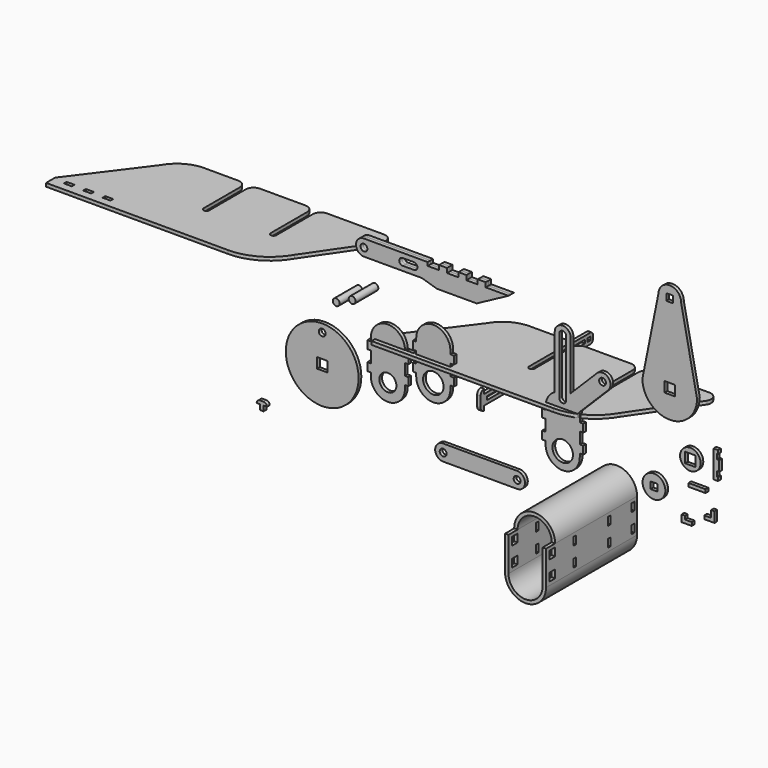
from build123d import *

# Parameters (mm, degrees)
F3_W      = 7
F3_H      = 3
F4_DEPTH  = 3
F2_W      = 7
F2_H      = 3
F5_DEPTH  = 3
F0_R      = 3
F6_DEPTH  = 3
F7_DEPTH  = 3
F8_R      = 9
F8_R_2    = 3
F9_DEPTH  = 3
F10_R     = 3
F11_DEPTH = 25
F12_R     = 3
F13_DEPTH = 25
F14_R     = 32
F14_W     = 9
F14_H     = 9
F14_R_2   = 3
F15_DEPTH = 3
F16_R     = 3
F17_DEPTH = 3
F18_R     = 10
F19_DEPTH = 100
F21_DEPTH = 100
F22_W     = 10
F22_H     = 18
F22_W_2   = 6
F22_H_2   = 7
F22_W_3   = 3
F23_DEPTH = 549.1479035941
F24_R     = 9
F25_DEPTH = 3
F1_R      = 7.5
F26_DEPTH = 3
F27_W     = 21
F27_H     = 3
F27_W_2   = 6
F27_W_3   = 18
F27_W_4   = 3
F28_DEPTH = 3
F29_R     = 3
F30_W     = 9
F30_H     = 9
F30_W_2   = 6
F30_H_2   = 6
F31_DEPTH = 3
F32_R     = 9
F32_W     = 9
F32_H     = 9
F33_DEPTH = 3
F35_DEPTH = 3
F36_DEPTH = 9
F38_DEPTH = 3
F40_W     = 3
F40_H     = 3
F41_DEPTH = 3
F43_DEPTH = 3
F45_DEPTH = 3
F46_W     = 15
F46_H     = 3
F47_DEPTH = 3
F48_R     = 10
F48_W     = 6
F48_H     = 6
F49_DEPTH = 3


# Not quite as in the source:
# - a feature names something its author has since deleted; it is built from what else it names


with BuildPart() as f4:
    # F3 (on Top) → F4 (new body)
    with BuildSketch(Plane.XY):
        with BuildLine():
            Line((-372.4580572146, 47.2241180668), (-372.4580572146, 37.2241180668))
            Line((-372.4580572146, 37.2241180668), (-212.4580572146, 37.2241180668))
            ThreePointArc((-212.4580572146, 37.2241180668), (-189.4580572146, 43.3869494928), (-172.6208886405, 60.2241180668))
            Line((-172.6208886405, 60.2241180668), (-137.4151172746, 111.7241180668))
            ThreePointArc((-137.4151172746, 111.7241180668), (-137.4151172746, 118.7241180668), (-143.4772951011, 122.2241180668))
            Line((-143.4772951011, 122.2241180668), (-193.4772951011, 122.2241180668))
            ThreePointArc((-193.4772951011, 122.2241180668), (-198.4270425694, 120.1738655351), (-200.4772951011, 115.2241180668))
            Line((-200.4772951011, 115.2241180668), (-200.4772951011, 75.2241180668))
            ThreePointArc((-200.4772951011, 75.2241180668), (-202.9772951011, 72.7241180668), (-205.4772951011, 75.2241180668))
            Line((-205.4772951011, 75.2241180668), (-205.4772951011, 115.2241180668))
            ThreePointArc((-205.4772951011, 115.2241180668), (-207.5275476328, 120.1738655351), (-212.4772951011, 122.2241180668))
            Line((-212.4772951011, 122.2241180668), (-252.4772951011, 122.2241180668))
            ThreePointArc((-252.4772951011, 122.2241180668), (-257.4270425694, 120.1738655351), (-259.4772951011, 115.2241180668))
            Line((-259.4772951011, 115.2241180668), (-259.4772951011, 75.2241180668))
            ThreePointArc((-259.4772951011, 75.2241180668), (-261.9772951011, 72.7241180668), (-264.4772951011, 75.2241180668))
            Line((-264.4772951011, 75.2241180668), (-264.4772951011, 115.2241180668))
            ThreePointArc((-264.4772951011, 115.2241180668), (-266.5275476328, 120.1738655351), (-271.4772951011, 122.2241180668))
            Line((-271.4772951011, 122.2241180668), (-301.4772951011, 122.2241180668))
            ThreePointArc((-301.4772951011, 122.2241180668), (-316.4772951011, 118.2048801804), (-327.4580572146, 107.2241180668))
            Line((-327.4580572146, 107.2241180668), (-372.4580572146, 47.2241180668))
        make_face()
        with Locations((-358.9580572146, 45.7241180668)):
            Rectangle(F3_W, F3_H, mode=Mode.SUBTRACT)
        with Locations((-341.9580572146, 45.7241180668)):
            Rectangle(F3_W, F3_H, mode=Mode.SUBTRACT)
        with Locations((-324.9580572146, 45.7241180668)):
            Rectangle(F3_W, F3_H, mode=Mode.SUBTRACT)
    extrude(amount=F4_DEPTH)


with BuildPart() as f5:
    # F2 (on Top) → F5 (new body)
    with BuildSketch(Plane.XY):
        with BuildLine():
            Line((-51.2112602569, 3.1967771862), (-51.2112602569, -6.8032228138))
            Line((-51.2112602569, -6.8032228138), (108.7887397431, -6.8032228138))
            ThreePointArc((108.7887397431, -6.8032228138), (131.7887397431, -0.6403913879), (148.6259083172, 16.1967771862))
            Line((148.6259083172, 16.1967771862), (183.8316796831, 67.6967771862))
            ThreePointArc((183.8316796831, 67.6967771862), (183.8316796831, 74.6967771862), (177.7695018566, 78.1967771862))
            Line((177.7695018566, 78.1967771862), (127.7695018566, 78.1967771862))
            ThreePointArc((127.7695018566, 78.1967771862), (122.8197543883, 76.1465246545), (120.7695018566, 71.1967771862))
            Line((120.7695018566, 71.1967771862), (120.7695018566, 31.1967771862))
            ThreePointArc((120.7695018566, 31.1967771862), (118.2695018566, 28.6967771862), (115.7695018566, 31.1967771862))
            Line((115.7695018566, 31.1967771862), (115.7695018566, 71.1967771862))
            ThreePointArc((115.7695018566, 71.1967771862), (113.7192493249, 76.1465246545), (108.7695018566, 78.1967771862))
            Line((108.7695018566, 78.1967771862), (68.7695018566, 78.1967771862))
            ThreePointArc((68.7695018566, 78.1967771862), (63.8197543883, 76.1465246545), (61.7695018566, 71.1967771862))
            Line((61.7695018566, 71.1967771862), (61.7695018566, 31.1967771862))
            ThreePointArc((61.7695018566, 31.1967771862), (59.2695018566, 28.6967771862), (56.7695018566, 31.1967771862))
            Line((56.7695018566, 31.1967771862), (56.7695018566, 71.1967771862))
            ThreePointArc((56.7695018566, 71.1967771862), (54.7192493249, 76.1465246545), (49.7695018566, 78.1967771862))
            Line((49.7695018566, 78.1967771862), (19.7695018566, 78.1967771862))
            ThreePointArc((19.7695018566, 78.1967771862), (4.7695018566, 74.1775392997), (-6.2112602569, 63.1967771862))
            Line((-6.2112602569, 63.1967771862), (-51.2112602569, 3.1967771862))
        make_face()
        with Locations((-37.7112602569, -1.3032228138)):
            Rectangle(F2_W, F2_H, mode=Mode.SUBTRACT)
        with Locations((-20.7112602569, -1.3032228138)):
            Rectangle(F2_W, F2_H, mode=Mode.SUBTRACT)
        with Locations((-3.7112602569, -1.3032228138)):
            Rectangle(F2_W, F2_H, mode=Mode.SUBTRACT)
    extrude(amount=F5_DEPTH)


with BuildPart() as f6:
    # F0 (on Front) → F6 (new body)
    with BuildSketch(Plane.XZ):
        with BuildLine():
            Line((-9.9334669923, 77.5954357982), (-60.9334669923, 77.5954357982))
            ThreePointArc((-60.9334669923, 77.5954357982), (-67.9334669923, 70.5954357982), (-60.9334669923, 63.5954357982))
            Line((-60.9334669923, 63.5954357982), (-9.9334669923, 63.5954357982))
            Line((-9.9334669923, 63.5954357982), (3.0665330077, 59.5954357982))
            Line((3.0665330077, 59.5954357982), (38.0665330077, 59.5954357982))
            Line((38.0665330077, 59.5954357982), (66.0665330077, 74.5954357982))
            Line((66.0665330077, 74.5954357982), (46.0665330077, 74.5954357982))
            Line((46.0665330077, 74.5954357982), (46.0665330077, 78.5954357982))
            Line((46.0665330077, 78.5954357982), (39.0665330077, 78.5954357982))
            Line((39.0665330077, 78.5954357982), (39.0665330077, 74.5954357982))
            Line((39.0665330077, 74.5954357982), (29.0665330077, 74.5954357982))
            Line((29.0665330077, 74.5954357982), (29.0665330077, 78.5954357982))
            Line((29.0665330077, 78.5954357982), (22.0665330077, 78.5954357982))
            Line((22.0665330077, 78.5954357982), (22.0665330077, 74.5954357982))
            Line((22.0665330077, 74.5954357982), (12.0665330077, 74.5954357982))
            Line((12.0665330077, 74.5954357982), (12.0665330077, 78.5954357982))
            Line((12.0665330077, 78.5954357982), (5.0665330077, 78.5954357982))
            Line((5.0665330077, 78.5954357982), (5.0665330077, 74.5954357982))
            Line((5.0665330077, 74.5954357982), (-4.9334669923, 74.5954357982))
            Line((-4.9334669923, 74.5954357982), (-4.9334669923, 77.5954357982))
            Line((-4.9334669923, 77.5954357982), (-9.9334669923, 77.5954357982))
        make_face()
        with Locations((-60.9334669923, 70.5954357982)):
            Circle(F0_R, mode=Mode.SUBTRACT)
        with BuildLine():
            ThreePointArc((-26.8621548395, 67.5954357982), (-29.9343144432, 70.5954357982), (-26.8621548395, 73.5954357982))
            Line((-26.8621548395, 73.5954357982), (-16.9334669923, 73.5954357982))
            ThreePointArc((-16.9334669923, 73.5954357982), (-13.9334669923, 70.5954357982), (-16.9334669923, 67.5954357982))
            Line((-16.9334669923, 67.5954357982), (-26.8621548395, 67.5954357982))
        make_face(mode=Mode.SUBTRACT)
    extrude(amount=F6_DEPTH)


with BuildPart() as f7:
    # F0 (on Front) → F7 (new body)
    with BuildSketch(Plane.XZ):
        with BuildLine():
            Line((-9.9334669923, 77.5954357982), (-60.9334669923, 77.5954357982))
            ThreePointArc((-60.9334669923, 77.5954357982), (-67.9334669923, 70.5954357982), (-60.9334669923, 63.5954357982))
            Line((-60.9334669923, 63.5954357982), (-9.9334669923, 63.5954357982))
            Line((-9.9334669923, 63.5954357982), (3.0665330077, 59.5954357982))
            Line((3.0665330077, 59.5954357982), (38.0665330077, 59.5954357982))
            Line((38.0665330077, 59.5954357982), (66.0665330077, 74.5954357982))
            Line((66.0665330077, 74.5954357982), (46.0665330077, 74.5954357982))
            Line((46.0665330077, 74.5954357982), (46.0665330077, 78.5954357982))
            Line((46.0665330077, 78.5954357982), (39.0665330077, 78.5954357982))
            Line((39.0665330077, 78.5954357982), (39.0665330077, 74.5954357982))
            Line((39.0665330077, 74.5954357982), (29.0665330077, 74.5954357982))
            Line((29.0665330077, 74.5954357982), (29.0665330077, 78.5954357982))
            Line((29.0665330077, 78.5954357982), (22.0665330077, 78.5954357982))
            Line((22.0665330077, 78.5954357982), (22.0665330077, 74.5954357982))
            Line((22.0665330077, 74.5954357982), (12.0665330077, 74.5954357982))
            Line((12.0665330077, 74.5954357982), (12.0665330077, 78.5954357982))
            Line((12.0665330077, 78.5954357982), (5.0665330077, 78.5954357982))
            Line((5.0665330077, 78.5954357982), (5.0665330077, 74.5954357982))
            Line((5.0665330077, 74.5954357982), (-4.9334669923, 74.5954357982))
            Line((-4.9334669923, 74.5954357982), (-4.9334669923, 77.5954357982))
            Line((-4.9334669923, 77.5954357982), (-9.9334669923, 77.5954357982))
        make_face()
        with Locations((-60.9334669923, 70.5954357982)):
            Circle(F0_R, mode=Mode.SUBTRACT)
        with BuildLine():
            ThreePointArc((-26.8621548395, 67.5954357982), (-29.9343144432, 70.5954357982), (-26.8621548395, 73.5954357982))
            Line((-26.8621548395, 73.5954357982), (-16.9334669923, 73.5954357982))
            ThreePointArc((-16.9334669923, 73.5954357982), (-13.9334669923, 70.5954357982), (-16.9334669923, 67.5954357982))
            Line((-16.9334669923, 67.5954357982), (-26.8621548395, 67.5954357982))
        make_face(mode=Mode.SUBTRACT)
    extrude(amount=-F7_DEPTH)


with BuildPart() as f9:
    # F8 (on Front) → F9 (new body)
    with BuildSketch(Plane.XZ):
        with BuildLine():
            Line((143.7687563849, 39.9497474683), (120.7185038532, 16.8994949366))
            Line((120.7185038532, 16.8994949366), (120.7185038532, 60))
            ThreePointArc((120.7185038532, 60), (113.7185038532, 67), (106.7185038532, 60))
            Line((106.7185038532, 60), (106.7185038532, 13.2664991614))
            ThreePointArc((106.7185038532, 13.2664991614), (100.8732712746, 7.7459666924), (98.7185038532, 0))
            Line((98.7185038532, 0), (98.7185038532, -3))
            Line((98.7185038532, -3), (95.7185038532, -3))
            Line((95.7185038532, -3), (95.7185038532, -10))
            Line((95.7185038532, -10), (98.7185038532, -10))
            Line((98.7185038532, -10), (98.7185038532, -20))
            Line((98.7185038532, -20), (95.7185038532, -20))
            Line((95.7185038532, -20), (95.7185038532, -27))
            Line((95.7185038532, -27), (98.7185038532, -27))
            Line((98.7185038532, -27), (98.7185038532, -30))
            ThreePointArc((98.7185038532, -30), (113.7185038532, -45), (128.7185038532, -30))
            Line((128.7185038532, -30), (128.7185038532, -27))
            Line((128.7185038532, -27), (131.7185038532, -27))
            Line((131.7185038532, -27), (131.7185038532, -20))
            Line((131.7185038532, -20), (128.7185038532, -20))
            Line((128.7185038532, -20), (128.7185038532, -10))
            Line((128.7185038532, -10), (131.7185038532, -10))
            Line((131.7185038532, -10), (131.7185038532, -3))
            Line((131.7185038532, -3), (128.7185038532, -3))
            Line((128.7185038532, -3), (128.7185038532, 0))
            ThreePointArc((128.7185038532, 0), (128.5502044438, 2.2406823939), (128.0490828412, 4.4310840513))
            Line((128.0490828412, 4.4310840513), (153.6682513215, 30.0502525317))
            ThreePointArc((153.6682513215, 30.0502525317), (153.6682513215, 39.9497474683), (143.7687563849, 39.9497474683))
        make_face()
        with Locations((113.7185038532, -30)):
            Circle(F8_R, mode=Mode.SUBTRACT)
        with BuildLine():
            ThreePointArc((110.7185038532, 60), (113.7185038532, 63), (116.7185038532, 60))
            Line((116.7185038532, 60), (116.7185038532, 10))
            ThreePointArc((116.7185038532, 10), (113.7185038532, 7), (110.7185038532, 10))
            Line((110.7185038532, 10), (110.7185038532, 60))
        make_face(mode=Mode.SUBTRACT)
        with Locations((148.7185038532, 35)):
            Circle(F8_R_2, mode=Mode.SUBTRACT)
    extrude(amount=F9_DEPTH)


with BuildPart() as f11:
    # F10 (on Front) → F11 (new body)
    with BuildSketch(Plane.XZ):
        with Locations((-67.738763988, 35.0489877164)):
            Circle(F10_R)
    extrude(amount=F11_DEPTH)


with BuildPart() as f13:
    # F12 (on Front) → F13 (new body)
    with BuildSketch(Plane.XZ):
        with Locations((-53.7285208702, 41.2954054773)):
            Circle(F12_R)
    extrude(amount=F13_DEPTH)


with BuildPart() as f15:
    # F14 (on Front) → F15 (new body)
    with BuildSketch(Plane.XZ):
        with Locations((-97.6346167383, -32)):
            Circle(F14_R)
        with Locations((-97.6346167383, -32)):
            Rectangle(F14_W, F14_H, mode=Mode.SUBTRACT)
        with Locations((-97.6346167383, -7)):
            Circle(F14_R_2, mode=Mode.SUBTRACT)
    extrude(amount=F15_DEPTH)


with BuildPart() as f17:
    # F16 (on Front) → F17 (new body)
    with BuildSketch(Plane.XZ):
        with BuildLine():
            Line((73.6428722739, -58.3517984152), (8.6428722739, -58.3517984152))
            ThreePointArc((8.6428722739, -58.3517984152), (1.6428722739, -65.3517984152), (8.6428722739, -72.3517984152))
            Line((8.6428722739, -72.3517984152), (73.6428722739, -72.3517984152))
            ThreePointArc((73.6428722739, -72.3517984152), (80.6428722739, -65.3517984152), (73.6428722739, -58.3517984152))
        make_face()
        with Locations((8.6428722739, -65.3517984152)):
            Circle(F16_R, mode=Mode.SUBTRACT)
        with Locations((73.6428722739, -65.3517984152)):
            Circle(F16_R, mode=Mode.SUBTRACT)
    extrude(amount=F17_DEPTH)


with BuildPart() as f19:
    # F18 (on Front) → F19 (new body)
    with BuildSketch(Plane.XZ):
        with Locations((-45.5094501376, -58.8990114629)):
            Circle(F18_R)
    extrude(amount=F19_DEPTH)


with BuildPart() as f21:
    # F20 (on Front) → F21 (new body)
    with BuildSketch(Plane.XZ):
        with BuildLine():
            ThreePointArc((176.6888463795, -45.6750293076), (158.6888463795, -27.6750293076), (140.6888463795, -45.6750293076))
            Line((140.6888463795, -45.6750293076), (140.6888463795, -75.6750293076))
            ThreePointArc((140.6888463795, -75.6750293076), (158.6888463795, -93.6750293076), (176.6888463795, -75.6750293076))
            Line((176.6888463795, -75.6750293076), (176.6888463795, -45.6750293076))
        make_face()
        with BuildLine():
            Line((173.6888463795, -45.6750293076), (173.6888463795, -75.6750293076))
            ThreePointArc((173.6888463795, -75.6750293076), (158.6888463795, -90.6750293076), (143.6888463795, -75.6750293076))
            Line((143.6888463795, -75.6750293076), (143.6888463795, -45.6750293076))
            ThreePointArc((143.6888463795, -45.6750293076), (158.6888463795, -30.6750293076), (173.6888463795, -45.6750293076))
        make_face(mode=Mode.SUBTRACT)
    extrude(amount=F21_DEPTH)


with BuildPart() as f23_tool:
    # F22 (on face) → F23 (new body, through all)
    with BuildSketch(Plane.YZ.offset(176.6888463795)):
        with Locations((-95, -36.6750293076)):
            Rectangle(F22_W, F22_H)
        with Locations((-93, -52.1750293076)):
            Rectangle(F22_W_2, F22_H_2)
        with Locations((-93, -69.1750293076)):
            Rectangle(F22_W_2, F22_H_2)
        with Locations((-4.5, -52.1750293076)):
            Rectangle(F22_W_3, F22_H_2)
        with Locations((-4.5, -69.1750293076)):
            Rectangle(F22_W_3, F22_H_2)
        with Locations((-68.5, -52.1750293076)):
            Rectangle(F22_W_3, F22_H_2)
        with Locations((-30.5, -52.1750293076)):
            Rectangle(F22_W_3, F22_H_2)
        with Locations((-68.5, -69.1750293076)):
            Rectangle(F22_W_3, F22_H_2)
        with Locations((-30.5, -69.1750293076)):
            Rectangle(F22_W_3, F22_H_2)
    extrude(amount=-F23_DEPTH)


with BuildPart() as f19_1:
    add(f19.part)

    # F23: cut by f23_tool
    add(f23_tool.part, mode=Mode.SUBTRACT)


with BuildPart() as f21_1:
    add(f21.part)

    # F23: cut by f23_tool
    add(f23_tool.part, mode=Mode.SUBTRACT)


with BuildPart() as f25:
    # F24 (on Front) → F25 (new body)
    with BuildSketch(Plane.XZ):
        with BuildLine():
            Line((15, 12.652173913), (15, 15.652173913))
            ThreePointArc((15, 15.652173913), (0, 30.652173913), (-15, 15.652173913))
            Line((-15, 15.652173913), (-15, 12.652173913))
            Line((-15, 12.652173913), (-18, 12.652173913))
            Line((-18, 12.652173913), (-18, 5.652173913))
            Line((-18, 5.652173913), (-15, 5.652173913))
            Line((-15, 5.652173913), (-15, -4.347826087))
            Line((-15, -4.347826087), (-18, -4.347826087))
            Line((-18, -4.347826087), (-18, -11.347826087))
            Line((-18, -11.347826087), (-15, -11.347826087))
            Line((-15, -11.347826087), (-15, -14.347826087))
            ThreePointArc((-15, -14.347826087), (0, -29.347826087), (15, -14.347826087))
            Line((15, -14.347826087), (15, -11.347826087))
            Line((15, -11.347826087), (18, -11.347826087))
            Line((18, -11.347826087), (18, -4.347826087))
            Line((18, -4.347826087), (15, -4.347826087))
            Line((15, -4.347826087), (15, 5.652173913))
            Line((15, 5.652173913), (18, 5.652173913))
            Line((18, 5.652173913), (18, 12.652173913))
            Line((18, 12.652173913), (15, 12.652173913))
        make_face()
        with Locations((0, -14.347826087)):
            Circle(F24_R, mode=Mode.SUBTRACT)
    extrude(amount=F25_DEPTH)


with BuildPart() as f26:
    # F1 (on Front) → F26 (new body)
    with BuildSketch(Plane.XZ):
        with BuildLine():
            Line((-24.9109024407, 0), (-24.9109024407, 3))
            ThreePointArc((-24.9109024407, 3), (-39.9109024407, 18), (-54.9109024407, 3))
            Line((-54.9109024407, 3), (-54.9109024407, 0))
            Line((-54.9109024407, 0), (-57.9109024407, 0))
            Line((-57.9109024407, 0), (-57.9109024407, -7))
            Line((-57.9109024407, -7), (-54.9109024407, -7))
            Line((-54.9109024407, -7), (-54.9109024407, -17))
            Line((-54.9109024407, -17), (-57.9109024407, -17))
            Line((-57.9109024407, -17), (-57.9109024407, -24))
            Line((-57.9109024407, -24), (-54.9109024407, -24))
            Line((-54.9109024407, -24), (-54.9109024407, -27))
            ThreePointArc((-54.9109024407, -27), (-39.9109024407, -42), (-24.9109024407, -27))
            Line((-24.9109024407, -27), (-24.9109024407, -24))
            Line((-24.9109024407, -24), (-21.9109024407, -24))
            Line((-21.9109024407, -24), (-21.9109024407, -17))
            Line((-21.9109024407, -17), (-24.9109024407, -17))
            Line((-24.9109024407, -17), (-24.9109024407, -7))
            Line((-24.9109024407, -7), (-21.9109024407, -7))
            Line((-21.9109024407, -7), (-21.9109024407, 0))
            Line((-21.9109024407, 0), (-24.9109024407, 0))
        make_face()
        with Locations((-39.9109024407, -27)):
            Circle(F1_R, mode=Mode.SUBTRACT)
    extrude(amount=F26_DEPTH)


with BuildPart() as f28:
    # F27 (on Right) → F28 (new body)
    with BuildSketch(Plane.YZ):
        with BuildLine():
            Line((168.6877954006, -43.0502752364), (49.1877954006, -43.0502752364))
            Line((49.1877954006, -43.0502752364), (49.1877954006, -39.0502752364))
            ThreePointArc((49.1877954006, -39.0502752364), (46.3593682759, -40.2218481116), (45.1877954006, -43.0502752364))
            Line((45.1877954006, -43.0502752364), (45.1877954006, -52.0502752364))
            ThreePointArc((45.1877954006, -52.0502752364), (46.3593682759, -54.8787023611), (49.1877954006, -56.0502752364))
            Line((49.1877954006, -56.0502752364), (49.1877954006, -52.0502752364))
            Line((49.1877954006, -52.0502752364), (168.6877954006, -52.0502752364))
            Line((168.6877954006, -52.0502752364), (168.6877954006, -43.0502752364))
        make_face()
        with Locations((62.6877954006, -47.5502752364)):
            Rectangle(F27_W, F27_H, mode=Mode.SUBTRACT)
        with Locations((104.1877954006, -47.5502752364)):
            Rectangle(F27_W_2, F27_H, mode=Mode.SUBTRACT)
        with Locations((150.6877954006, -47.5502752364)):
            Rectangle(F27_W_3, F27_H, mode=Mode.SUBTRACT)
        with Locations((164.1877954006, -47.5502752364)):
            Rectangle(F27_W_4, F27_H, mode=Mode.SUBTRACT)
    extrude(amount=F28_DEPTH)

    # F29
    f29_edges = [f28.edges().sort_by_distance(p)[0] for p in [
        (1.5, 168.687795, -43.050275),
        (1.5, 168.687795, -52.050275),
    ]]
    fillet(f29_edges, radius=F29_R)


with BuildPart() as f31:
    # F30 (on Front) → F31 (new body)
    with BuildSketch(Plane.XZ):
        with BuildLine():
            Line((197.7664567232, 118.7906804383), (183.7664567232, 48.7906804383))
            ThreePointArc((183.7664567232, 48.7906804383), (207.7664567232, 24.7906804383), (231.7664567232, 48.7906804383))
            Line((231.7664567232, 48.7906804383), (217.7664567232, 118.7906804383))
            ThreePointArc((217.7664567232, 118.7906804383), (207.7664567232, 128.7906804383), (197.7664567232, 118.7906804383))
        make_face()
        with Locations((207.7664567232, 48.7906804383)):
            Rectangle(F30_W, F30_H, mode=Mode.SUBTRACT)
        with Locations((207.7664567232, 118.7906804383)):
            Rectangle(F30_W_2, F30_H_2, mode=Mode.SUBTRACT)
    extrude(amount=F31_DEPTH)


with BuildPart() as f33:
    # F32 (on Front) → F33 (new body)
    with BuildSketch(Plane.XZ):
        with Locations((225.8719205856, 0)):
            Circle(F32_R)
        with Locations((225.8719205856, 0)):
            Rectangle(F32_W, F32_H, mode=Mode.SUBTRACT)
    extrude(amount=F33_DEPTH)


with BuildPart() as f35:
    # F34 (on Front) → F35 (new body)
    with BuildSketch(Plane.XZ):
        Polygon((249.2403327227, 7.5919592045), (249.2403327227, 12.0919592045), (250.2403327227, 12.0919592045), (250.2403327227, 15.0919592045), (246.2403327227, 15.0919592045), (246.2403327227, -8.9080407955), (250.2403327227, -8.9080407955), (250.2403327227, -5.9080407955), (249.2403327227, -5.9080407955), (249.2403327227, -1.4080407955), (251.2403327227, -1.4080407955), (251.2403327227, 7.5919592045), align=None)
    extrude(amount=F35_DEPTH)


with BuildPart() as f36:
    # F27 (on Right) → F36 (new body)
    with BuildSketch(Plane.YZ):
        with Locations((104.1877954006, -47.5502752364)):
            Rectangle(F27_W_2, F27_H)
    extrude(amount=F36_DEPTH)


with BuildPart() as f38:
    # F37 (on Front) → F38 (new body)
    with BuildSketch(Plane.XZ):
        with BuildLine():
            Line((-155.1654338837, -80.3057419062), (-152.1654338837, -80.3057419062))
            Line((-152.1654338837, -80.3057419062), (-152.1654338837, -84.8057419062))
            Line((-152.1654338837, -84.8057419062), (-149.1654338837, -84.8057419062))
            Line((-149.1654338837, -84.8057419062), (-149.1654338837, -80.3057419062))
            Line((-149.1654338837, -80.3057419062), (-146.1654338837, -80.3057419062))
            ThreePointArc((-146.1654338837, -80.3057419062), (-147.0441135401, -78.1844215626), (-149.1654338837, -77.3057419062))
            Line((-149.1654338837, -77.3057419062), (-152.1654338837, -77.3057419062))
            ThreePointArc((-152.1654338837, -77.3057419062), (-154.2867542272, -78.1844215626), (-155.1654338837, -80.3057419062))
        make_face()
    extrude(amount=F38_DEPTH)


with BuildPart() as f41:
    # F40 (on Right) → F41 (new body)
    with BuildSketch(Plane.YZ):
        with BuildLine():
            Line((79.3230089621, -16.1746714419), (79.3230089621, -13.1746714419))
            ThreePointArc((79.3230089621, -13.1746714419), (77.2016886185, -14.0533510983), (76.3230089621, -16.1746714419))
            Line((76.3230089621, -16.1746714419), (76.3230089621, -22.1746714419))
            ThreePointArc((76.3230089621, -22.1746714419), (77.2016886185, -24.2959917854), (79.3230089621, -25.1746714419))
            Line((79.3230089621, -25.1746714419), (79.3230089621, -22.1746714419))
            Line((79.3230089621, -22.1746714419), (98.8230089621, -22.1746714419))
            ThreePointArc((98.8230089621, -22.1746714419), (99.8836691339, -21.7353316136), (100.3230089621, -20.6746714419))
            Line((100.3230089621, -20.6746714419), (100.3230089621, -17.6746722149))
            ThreePointArc((100.3230089621, -17.6746722149), (99.8836694072, -16.6140115434), (98.8230089621, -16.1746714419))
            Line((98.8230089621, -16.1746714419), (79.3230089621, -16.1746714419))
        make_face()
        with Locations((83.8230089621, -19.1746715626)):
            Rectangle(F40_W, F40_H, mode=Mode.SUBTRACT)
        with Locations((95.8230089621, -19.1746717559)):
            Rectangle(F40_W, F40_H, mode=Mode.SUBTRACT)
    extrude(amount=F41_DEPTH)


with BuildPart() as f43:
    # F42 (on Front) → F43 (new body)
    with BuildSketch(Plane.XZ):
        Polygon((221.1307316584, -45.0849015334), (218.1307316584, -45.0849015334), (218.1307316584, -51.0849015334), (227.1307316584, -51.0849015334), (227.1307316584, -48.0849015334), (221.1307316584, -48.0849015334), align=None)
    extrude(amount=F43_DEPTH)


with BuildPart() as f45:
    # F44 (on Front) → F45 (new body)
    with BuildSketch(Plane.XZ):
        Polygon((238.1164150238, -39.2968996763), (238.1164150238, -42.2968996763), (247.1164150238, -42.2968996763), (247.1164150238, -33.2968996763), (244.1164150238, -33.2968996763), (244.1164150238, -39.2968996763), align=None)
    extrude(amount=F45_DEPTH)


with BuildPart() as f47:
    # F46 (on Front) → F47 (new body)
    with BuildSketch(Plane.XZ):
        with Locations((231.7560386658, -20.2369310558)):
            Rectangle(F46_W, F46_H)
    extrude(amount=F47_DEPTH)


with BuildPart() as f49:
    # F48 (on Front) → F49 (new body)
    with BuildSketch(Plane.XZ):
        with Locations((193.9209638834, -31.3312248588)):
            Circle(F48_R)
        with Locations((193.9209638834, -31.3312248588)):
            Rectangle(F48_W, F48_H, mode=Mode.SUBTRACT)
    extrude(amount=F49_DEPTH)


solid = Compound([f4.part, f5.part, f6.part, f7.part, f9.part, f11.part, f13.part, f15.part, f17.part, f21_1.part, f25.part, f26.part, f28.part, f31.part, f33.part, f35.part, f36.part, f38.part, f41.part, f43.part, f45.part, f47.part, f49.part])
